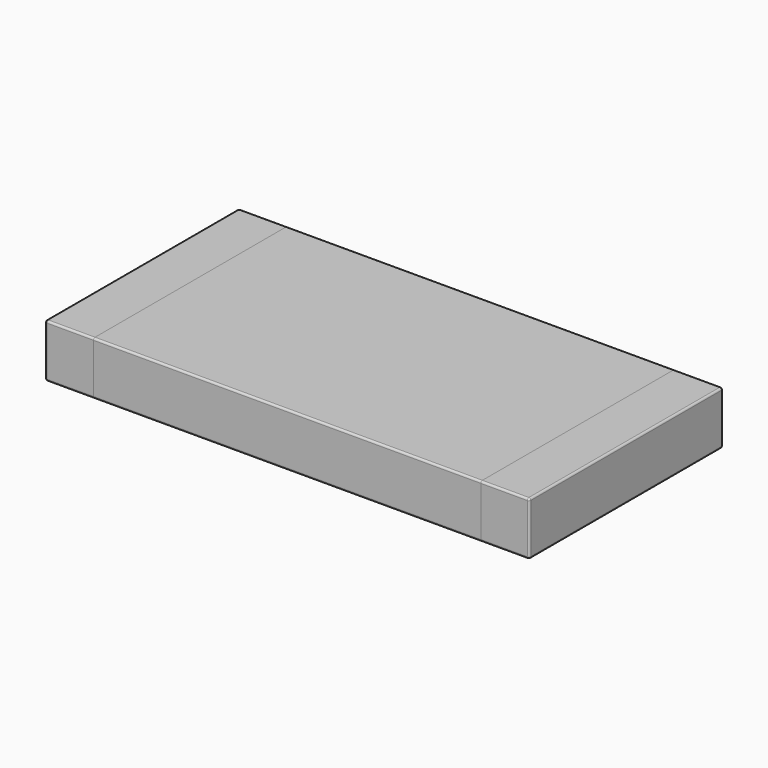
from build123d import *

# Parameters (mm, degrees)
F2_W     = 4
F2_H     = 2.5
F3_DEPTH = 0.53
F2_W_2   = 0.5
F4_DEPTH = 0.55
F5_DEPTH = 0.55
F6_DEPTH = 0.02
F7_R     = 0.01999
F7_2_R   = 0.01999
F7_3_R   = 0.01999
F7_4_R   = 0.01999


# Not quite as in the source:
# - a fillet or chamfer is up to 0.001 mm smaller than in the source, because OpenCascade refuses the exact size


with BuildPart() as f3:
    # F2 (on Top) → F3 (new body)
    with BuildSketch(Plane.XY):
        Rectangle(F2_W, F2_H)
    extrude(amount=F3_DEPTH)


with BuildPart() as f4:
    # F2 (on Top) → F4 (new body)
    with BuildSketch(Plane.XY):
        with Locations((-2.25, 0)):
            Rectangle(F2_W_2, F2_H)
    extrude(amount=F4_DEPTH)

    # F7 (radius 0.02 in the source; OpenCascade refuses exactly that, so slightly less here)
    f7_edges = [f4.edges().sort_by_distance(p)[0] for p in [
        (-2.25, -1.25, 0.55),
        (-2.5, 1.25, 0.275),
        (-2.5, -1.25, 0.275),
        (-2.5, 0, 0),
        (-2.5, 0, 0.55),
        (-2.25, 1.25, 0.55),
        (-2.25, 1.25, 0),
        (-2.25, -1.25, 0),
    ]]
    fillet(f7_edges, radius=F7_R)


with BuildPart() as f5:
    # F2 (on Top) → F5 (new body)
    with BuildSketch(Plane.XY):
        with Locations((2.25, 0)):
            Rectangle(F2_W_2, F2_H)
    extrude(amount=F5_DEPTH)

    # F7#2 (radius 0.02 in the source; OpenCascade refuses exactly that, so slightly less here)
    f7_2_edges = [f5.edges().sort_by_distance(p)[0] for p in [
        (2.25, -1.25, 0.55),
        (2.5, -1.25, 0.275),
        (2.5, 1.25, 0.275),
        (2.5, 0, 0),
        (2.5, 0, 0.55),
        (2.25, 1.25, 0.55),
        (2.25, 1.25, 0),
        (2.25, -1.25, 0),
    ]]
    fillet(f7_2_edges, radius=F7_2_R)


with BuildPart() as f6:
    # F6 (new): a face of the model
    f6_faces = [f3.part.faces().sort_by_distance(p)[0] for p in [
        (0, 0, 0.53),
    ]]
    extrude(f6_faces, amount=F6_DEPTH)

    # F7#4 (radius 0.02 in the source; OpenCascade refuses exactly that, so slightly less here)
    f7_4_edges = [f6.edges().sort_by_distance(p)[0] for p in [
        (0, -1.25, 0.55),
        (0, 1.25, 0.55),
    ]]
    fillet(f7_4_edges, radius=F7_4_R)


with BuildPart() as f3_1:
    add(f3.part)

    # F7#3 (radius 0.02 in the source; OpenCascade refuses exactly that, so slightly less here)
    f7_3_edges = [f3_1.edges().sort_by_distance(p)[0] for p in [
        (0, 1.25, 0),
        (0, -1.25, 0),
    ]]
    fillet(f7_3_edges, radius=F7_3_R)


solid = Compound([f4.part, f5.part, f6.part, f3_1.part])
